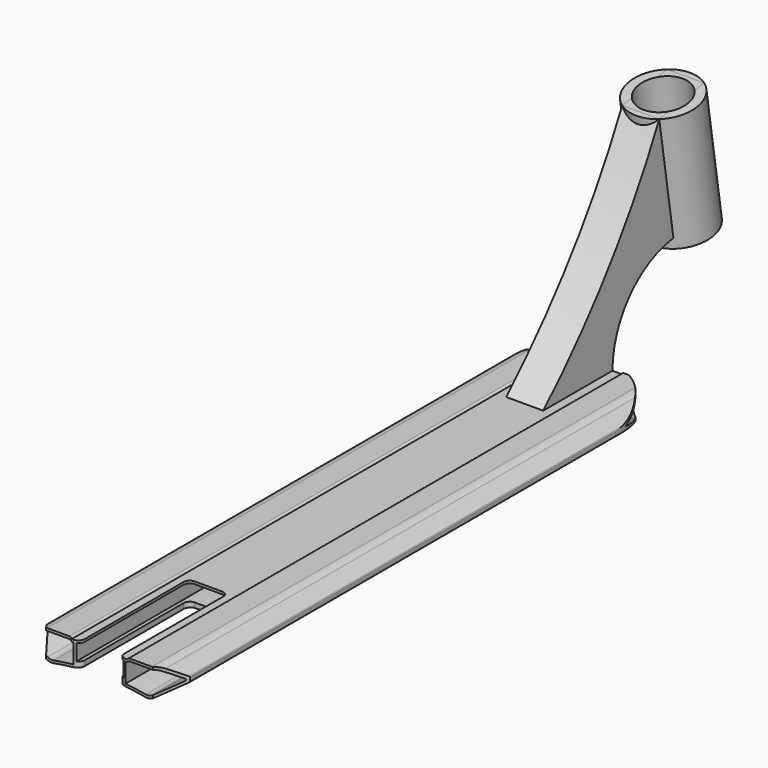
from build123d import *

# Parameters (mm, degrees)
F1_DEPTH       = 250
F2_W           = 38
F2_H           = 13
F3_DEPTH       = 500.001
F4_T1_DEPTH    = 509.3674969976
F5_R           = 9
F6_R           = 1
F8_DEPTH       = 500.001
F10_DEPTH      = 8.4253865001
F10_DEPTH_BACK = 15.0949186811
F12_DEPTH      = 15
F13_R          = 27.5
F14_DEPTH      = 100
F16_D          = 40
F18_DEPTH      = 8.4253866128
F18_DEPTH_BACK = 181.6948592657
F19_T1_DEPTH   = 2
F19_T6_DEPTH   = 16.7634824315
F19_S7_R       = 200
F19_T8_DEPTH   = 11
F19_T12_DEPTH  = 16.7634824315
F19_S13_R      = 200
F19_T14_DEPTH  = 11
F19_T15_DEPTH  = 27
F19_T17_DEPTH  = 29.2634824315


# Not quite as in the source:
# - a fillet or chamfer that OpenCascade refuses, or shapes differently, is made with other operations: its cross-section is extruded or revolved along the edge and cut away or added


with BuildPart() as f1:
    # F0 (on Front) → F1 (new body, symmetric)
    with BuildSketch(Plane.XZ):
        with BuildLine():
            Line((22.5, 13.7939186811), (0, 13.7939186811))
            Line((0, 13.7939186811), (-22.5, 13.7939186811))
            Line((-22.5, 13.7939186811), (-22.5, 15.0939186811))
            Line((-22.5, 15.0939186811), (-45.5824640741, 15.0939186811))
            Line((-45.5824640741, 15.0939186811), (-57.5, 5.0939186811))
            Line((-57.5, 5.0939186811), (-57.5, 1.0939186811))
            Line((-57.5, 1.0939186811), (-40.1794919243, -8.9060813189))
            ThreePointArc((-40.1794919243, -8.9060813189), (0, -4.8285364604), (40.1794919243, -8.9060813189))
            Line((40.1794919243, -8.9060813189), (57.5, 1.0939186811))
            Line((57.5, 1.0939186811), (57.5, 5.0939186811))
            Line((57.5, 5.0939186811), (45.5824640741, 15.0939186811))
            Line((45.5824640741, 15.0939186811), (22.5, 15.0939186811))
            Line((22.5, 15.0939186811), (22.5, 13.7939186811))
        make_face()
    extrude(amount=F1_DEPTH, both=True)

    # F2 (on face) → F3 (cut, through all)
    with BuildSketch(Plane.XZ.offset(250)):
        with Locations((0, 5.2939186811)):
            Rectangle(F2_W, F2_H)
    extrude(amount=-F3_DEPTH, mode=Mode.SUBTRACT)

    # F4: fillet of radius 2 on 2 edges, made by hand

    # F4_s2 → F4_t1 (cut)
    with BuildSketch(Plane.XZ.offset(-254.6837484988)):
        with BuildLine():
            ThreePointArc((24.3734993995, 15.0939186811), (23.2333239744, 14.7370863537), (22.5, 13.7939186811))
            Line((22.5, 13.7939186811), (22.5, 15.0939186811))
            Line((22.5, 15.0939186811), (24.3734993995, 15.0939186811))
        make_face()
        with BuildLine():
            ThreePointArc((-24.3734993995, 15.0939186811), (-23.2333239744, 14.7370863537), (-22.5, 13.7939186811))
            Line((-22.5, 13.7939186811), (-22.5, 15.0939186811))
            Line((-22.5, 15.0939186811), (-24.3734993995, 15.0939186811))
        make_face()
    extrude(amount=F4_T1_DEPTH, mode=Mode.SUBTRACT)

    # F5
    f5_edges = [f1.edges().sort_by_distance(p)[0] for p in [
        (45.582464, 0, 15.093919),
        (-45.582464, 0, 15.093919),
        (-40.179492, 0, -8.906081),
        (40.179492, 0, -8.906081),
    ]]
    fillet(f5_edges, radius=F5_R)

    # F6
    f6_edges = [f1.edges().sort_by_distance(p)[0] for p in [
        (57.5, 0, 1.093919),
        (57.5, 0, 5.093919),
        (-57.5, 0, 5.093919),
        (-57.5, 0, 1.093919),
    ]]
    fillet(f6_edges, radius=F6_R)

    # F7 (on face) → F8 (cut, through all)
    with BuildSketch(Plane.XZ.offset(250)):
        with BuildLine():
            Line((-55.6135241478, 2.3141624168), (-42.1022690923, -5.4865643266))
            ThreePointArc((-42.1022690923, -5.4865643266), (-39.7790673433, -6.3247593796), (-37.3093701274, -6.3039513313))
            ThreePointArc((-37.3093701274, -6.3039513313), (-29.1789785809, -4.9471035834), (-21, -3.9230860615))
            Line((-21, -3.9230860615), (-21, 11.7939186811))
            Line((-21, 11.7939186811), (-22.6125713953, 11.7939186811))
            ThreePointArc((-22.6125713953, 11.7939186811), (-23.3458953697, 12.7370863537), (-24.4860707948, 13.0939186811))
            Line((-24.4860707948, 13.0939186811), (-42.3067319657, 13.0939186811))
            ThreePointArc((-42.3067319657, 13.0939186811), (-44.7008729689, 12.6717670266), (-46.8062452335, 11.456229783))
            Line((-46.8062452335, 11.456229783), (-55.7563117574, 3.9462322637))
            ThreePointArc((-55.7563117574, 3.9462322637), (-56.1097188459, 3.0930320778), (-55.6135241478, 2.3141624168))
        make_face()
        with BuildLine():
            ThreePointArc((21, -3.9230860615), (29.1789785809, -4.9471035834), (37.3093701274, -6.3039513313))
            ThreePointArc((37.3093701274, -6.3039513313), (39.7790673433, -6.3247593796), (42.1022690923, -5.4865643266))
            Line((42.1022690923, -5.4865643266), (55.6135241478, 2.3141624168))
            ThreePointArc((55.6135241478, 2.3141624168), (56.1097188459, 3.0930320778), (55.7563117574, 3.9462322637))
            Line((55.7563117574, 3.9462322637), (46.8062452335, 11.456229783))
            ThreePointArc((46.8062452335, 11.456229783), (44.7008729689, 12.6717670266), (42.3067319657, 13.0939186811))
            Line((42.3067319657, 13.0939186811), (24.4860707948, 13.0939186811))
            ThreePointArc((24.4860707948, 13.0939186811), (23.3458953697, 12.7370863537), (22.6125713953, 11.7939186811))
            Line((22.6125713953, 11.7939186811), (21, 11.7939186811))
            Line((21, 11.7939186811), (21, -3.9230860615))
        make_face()
    extrude(amount=-F8_DEPTH, mode=Mode.SUBTRACT)

    # F9 (on Top) → F10 (cut, two sides)
    with BuildSketch(Plane.XY) as f10_sk:
        with BuildLine():
            ThreePointArc((-57.5, 200), (0, 257.5), (57.5, 200))
            Line((57.5, 200), (57.5, 280))
            Line((57.5, 280), (-57.5, 280))
            Line((-57.5, 280), (-57.5, 200))
        make_face()
    extrude(amount=-F10_DEPTH, mode=Mode.SUBTRACT)
    extrude(f10_sk.sketch, amount=F10_DEPTH_BACK, mode=Mode.SUBTRACT)

    # F11 (on Right) → F12 (join, symmetric)
    with BuildSketch(Plane.YZ):
        with BuildLine():
            ThreePointArc((297.3819995028, 173.7939186811), (245.9666940414, 88.4561965341), (180, 13.7939186811))
            Line((180, 13.7939186811), (250, 13.7939186811))
            ThreePointArc((250, 13.7939186811), (267.6550746197, 60.2698133678), (311.7145367693, 83.3018398057))
            Line((311.7145367693, 83.3018398057), (313.0254460068, 75.0250846216))
            Line((313.0254460068, 75.0250846216), (358.4591096742, 82.2210700135))
            Line((358.4591096742, 82.2210700135), (342.8156631702, 180.989904073))
            Line((342.8156631702, 180.989904073), (297.3819995028, 173.7939186811))
        make_face()
    extrude(amount=F12_DEPTH, both=True)

    # F13 (on face) → F14 (join, through all)
    with BuildSketch(Plane(origin=(0, -19.5751816724, 123.5928329339), x_dir=(1, 0, 0), z_dir=(0, -0.156434465, 0.9876883406))):
        with Locations((0, 343.9080923079)):
            Circle(F13_R)
    extrude(amount=-F14_DEPTH)

    # F16 (through all)
    with Locations(Plane(origin=(0, -19.5751816724, 123.5928329339), x_dir=(1, 0, 0), z_dir=(0, -0.156434465, 0.9876883406))):
        with Locations((0, 343.9080923079)):
            Hole(F16_D / 2)

    # F17 (on Top) → F18 (cut, two sides)
    with BuildSketch(Plane.XY) as f18_sk:
        Polygon((-43.2975540478, -250), (-68, -216), (-68, -346), (68, -346), (68, -216), (43.2975540478, -250), (16, -250), (16, -140), (-16, -140), (-16, -250), align=None)
    extrude(amount=-F18_DEPTH, mode=Mode.SUBTRACT)
    extrude(f18_sk.sketch, amount=F18_DEPTH_BACK, mode=Mode.SUBTRACT)

    # F19: fillet of radius 5 on 8 edges, made by hand

    # F19_s2 → F19_t1 (join)
    with BuildSketch(Plane.XY.offset(11.7939186811)):
        with BuildLine():
            ThreePointArc((-11, -140), (-14.5355339059, -141.4644660941), (-16, -145))
            Line((-16, -145), (-16, -140))
            Line((-16, -140), (-11, -140))
        make_face()
        with BuildLine():
            ThreePointArc((16, -145), (14.5355339059, -141.4644660941), (11, -140))
            Line((11, -140), (16, -140))
            Line((16, -140), (16, -145))
        make_face()
    extrude(amount=F19_T1_DEPTH)


with BuildPart() as f19_tool4:
    # F19_s5 → F19_t6 (new body)
    with BuildSketch(Plane.XY.offset(-1.2060813189)):
        with BuildLine():
            ThreePointArc((-16, -145), (-14.5355339059, -141.4644660941), (-11, -140))
            Line((-11, -140), (-16, -140))
            Line((-16, -140), (-16, -145))
        make_face()
    extrude(amount=-F19_T6_DEPTH)

    # F19_s7 → F19_t8 (cut, symmetric)
    with BuildSketch(Plane.XZ.offset(142.5)):
        with Locations((0, -204.8285364604)):
            Circle(F19_S7_R)
    extrude(amount=F19_T8_DEPTH, both=True, mode=Mode.SUBTRACT)


with BuildPart() as f1_1:
    add(f1.part)

    # F19_t3: union F19_tool4
    add(f19_tool4.part)


with BuildPart() as f19_tool10:
    # F19_s11 → F19_t12 (new body)
    with BuildSketch(Plane.XY.offset(-17.9695637504)):
        with BuildLine():
            ThreePointArc((11, -140), (14.5355339059, -141.4644660941), (16, -145))
            Line((16, -145), (16, -140))
            Line((16, -140), (11, -140))
        make_face()
    extrude(amount=F19_T12_DEPTH)

    # F19_s13 → F19_t14 (cut, symmetric)
    with BuildSketch(Plane.XZ.offset(142.5)):
        with Locations((0, -204.8285364604)):
            Circle(F19_S13_R)
    extrude(amount=F19_T14_DEPTH, both=True, mode=Mode.SUBTRACT)


with BuildPart() as f1_2:
    add(f1_1.part)

    # F19_t9: union F19_tool10
    add(f19_tool10.part)

    # F19_s16 → F19_t15 (cut)
    with BuildSketch(Plane.XY.offset(-0.7060813189)):
        with BuildLine():
            ThreePointArc((-21, -250), (-17.4644660941, -248.5355339059), (-16, -245))
            Line((-16, -245), (-16, -250))
            Line((-16, -250), (-21, -250))
        make_face()
        with BuildLine():
            ThreePointArc((21, -250), (17.4644660941, -248.5355339059), (16, -245))
            Line((16, -245), (16, -250))
            Line((16, -250), (21, -250))
        make_face()
    extrude(amount=F19_T15_DEPTH, mode=Mode.SUBTRACT)

    # F19_s18 → F19_t17 (cut)
    with BuildSketch(Plane.XY.offset(-17.9695637504)):
        with BuildLine():
            ThreePointArc((21, -250), (17.4644660941, -248.5355339059), (16, -245))
            Line((16, -245), (16, -250))
            Line((16, -250), (21, -250))
        make_face()
        with BuildLine():
            ThreePointArc((-21, -250), (-17.4644660941, -248.5355339059), (-16, -245))
            Line((-16, -245), (-16, -250))
            Line((-16, -250), (-21, -250))
        make_face()
    extrude(amount=F19_T17_DEPTH, mode=Mode.SUBTRACT)


solid = f1_2.part
